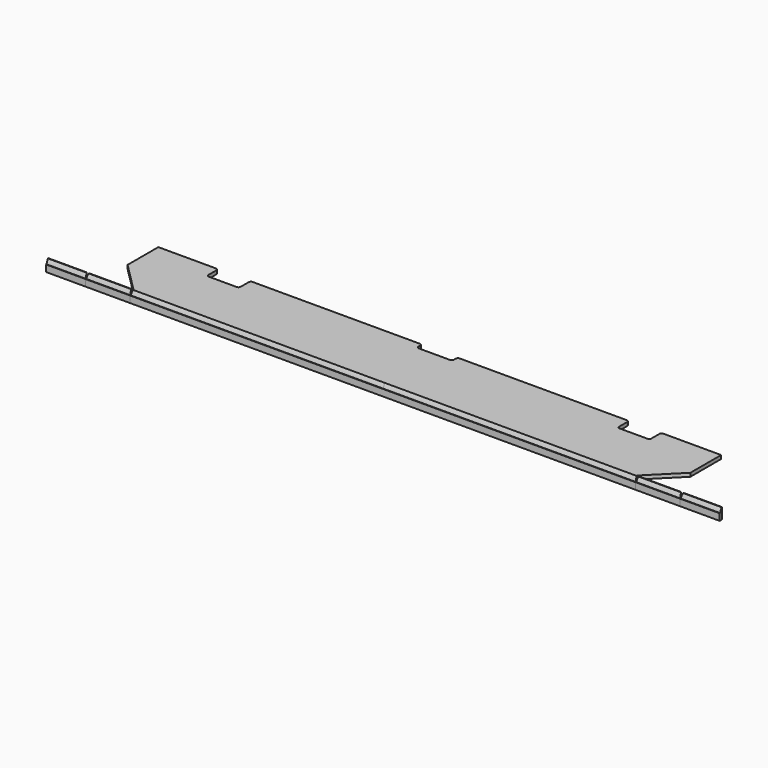
from build123d import *

# Parameters (mm, degrees)
F3_DEPTH      = 10.16
F4_W          = 2032
F4_H          = 7.9375
F5_DEPTH      = 57.15
F7_DEPTH      = 1016.001
F7_DEPTH_BACK = 1016.001
F8_W          = 7.9375
F8_H          = 25.4
F9_DEPTH      = 2032.0010001
F10_W         = 52.698585695
F10_H         = 7.9375
F11_DEPTH     = 31.7510001
F12_W         = 92.075
F12_H         = 41.275
F12_W_2       = 101.6
F12_H_2       = 19.05
F13_DEPTH     = 31.7510001
F14_R         = 6.35


# Not quite as in the source:
# - a variable given as a bare number and used for a length is read in inches; the dataset says mm whatever the document's units were


with BuildPart() as f3:
    # F2 (on Top) → F3 (new body)
    with BuildSketch(Plane.XY):
        Polygon((804.8625, 0), (-804.8625, 0), (-804.8625, -109.9500668498), (-719.5500668498, -195.2625), (719.5500668498, -195.2625), (804.8625, -109.9500668498), align=None)
    extrude(amount=-F3_DEPTH)

    # F12 (on face) → F13 (cut, through all)
    with BuildSketch(Plane.XY):
        with Locations((-587.375, -20.6375)):
            Rectangle(F12_W, F12_H)
        with Locations((0, -9.525)):
            Rectangle(F12_W_2, F12_H_2)
        with Locations((587.375, -20.6375)):
            Rectangle(F12_W, F12_H)
    extrude(amount=-F13_DEPTH, mode=Mode.SUBTRACT)

    # F14
    f14_edges = [f3.edges().sort_by_distance(p)[0] for p in [
        (-633.4125, 0, -5.08),
        (-633.4125, -41.275, -5.08),
        (-541.3375, -41.275, -5.08),
        (-541.3375, 0, -5.08),
        (-50.8, -19.05, -5.08),
        (-50.8, 0, -5.08),
        (50.8, 0, -5.08),
        (50.8, -19.05, -5.08),
        (633.4125, -41.275, -5.08),
        (633.4125, 0, -5.08),
        (541.3375, -41.275, -5.08),
        (541.3375, 0, -5.08),
    ]]
    fillet(f14_edges, radius=F14_R)


with BuildPart() as f5:
    # F4 (on face) → F5 (new body)
    with BuildSketch(Plane.XY):
        with Locations((0, -199.23125)):
            Rectangle(F4_W, F4_H)
    extrude(amount=-F5_DEPTH)

    # F6 (on Right) → F7 (cut, two sides)
    with BuildSketch(Plane.YZ) as f7_sk:
        with BuildLine():
            Line((-203.2, -12.7), (-201.7, -12.7))
            add(Edge.make_bspline(
                [(-196.7625, 0), (-196.8148604761, -0.3804030605), (-197.1200745243, -1.3902041101), (-198.7386405945, -4.2395784301), (-201.6317836716, -10.8737146377), (-201.7, -12.7)],
                knots=[0, 0, 0, 0, 0.1863946303, 0.5014086831, 1, 1, 1, 1], degree=3))
            Line((-196.7625, 0), (-203.2, 0))
            Line((-203.2, 0), (-203.2, -12.7))
        make_face()
    extrude(amount=-F7_DEPTH, mode=Mode.SUBTRACT)
    extrude(f7_sk.sketch, amount=F7_DEPTH_BACK, mode=Mode.SUBTRACT)

    # F8 (on face) → F9 (cut, through all)
    with BuildSketch(Plane.YZ.offset(1016)):
        with Locations((-199.23125, -44.45)):
            Rectangle(F8_W, F8_H)
    extrude(amount=-F9_DEPTH, mode=Mode.SUBTRACT)

    # F10 (on face) → F11 (cut, through all)
    with BuildSketch(Plane.XY):
        Polygon((-722.8378870012, -203.2), (-719.5500668498, -195.2625), (-726.1257071525, -195.2625), align=None)
        Polygon((-850.0635273039, -203.2), (-846.7757071525, -195.2625), (-853.3513474552, -195.2625), align=None)
        Polygon((726.1257071525, -195.2625), (719.5500668498, -195.2625), (722.8378870012, -203.2), align=None)
        Polygon((853.3513474552, -195.2625), (846.7757071525, -195.2625), (850.0635273039, -203.2), align=None)
        with Locations((-989.6507071525, -199.23125)):
            Rectangle(F10_W, F10_H)
        with Locations((989.6507071525, -199.23125)):
            Rectangle(F10_W, F10_H)
    extrude(amount=-F11_DEPTH, mode=Mode.SUBTRACT)


solid = Compound([f3.part, f5.part])
